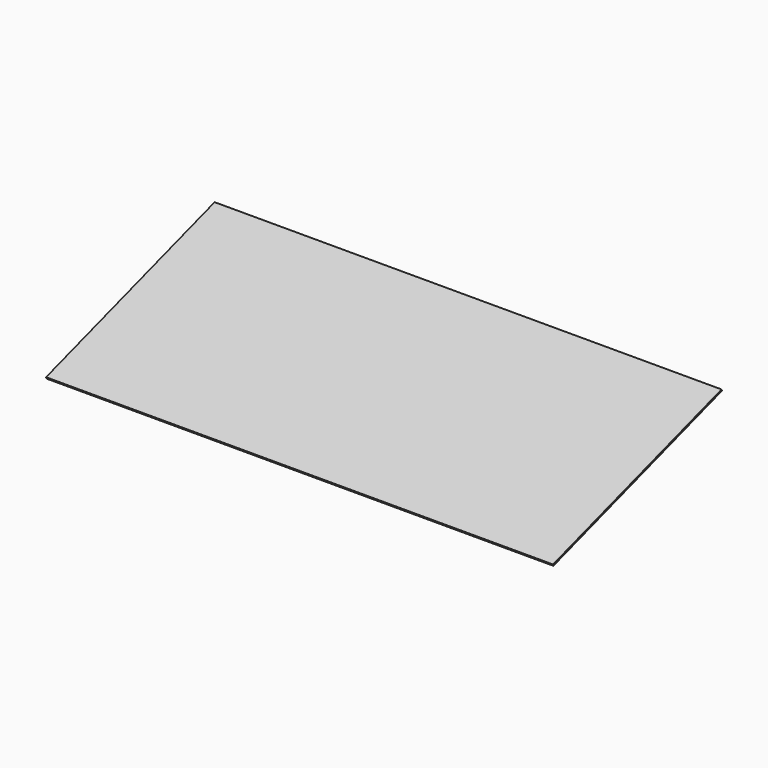
from build123d import *

# Parameters (mm, degrees)
F1_DEPTH = 550
F2_W     = 37.5
F2_H     = 447.9229075255
F3_DEPTH = 25


# Not quite as in the source:
# - a feature names something its author has since deleted; it is built from what else it names


with BuildPart() as f1:
    # F0 (on Right) → F1 (new body, symmetric)
    with BuildSketch(Plane.YZ):
        Polygon((1854.2745751406, 569.7310398559), (2042.2745751406, 630.8159427477), (2041.3475241575, 633.6691122966), (1853.3475241575, 572.5842094048), align=None)
        Polygon((2041.3475241575, 633.6691122966), (2042.2745751406, 630.8159427477), (2092.2745751406, 647.0619275593), (2091.3475241575, 649.9150971082), align=None)
        Polygon((2091.3475241575, 649.9150971082), (2092.2745751406, 647.0619275593), (2280.2745751406, 708.1468304511), (2279.3475241575, 711), align=None)
    extrude(amount=F1_DEPTH, both=True)

    # F2 (on face) → F3 (cut)
    with BuildSketch(Plane(origin=(0, 8.7006633238, -26.7778882743), x_dir=(1, 0, 0), z_dir=(0, -0.3090169944, 0.9510565163))):
        with Locations((-531.25, 2163.5379449891)):
            Rectangle(F2_W, F2_H)
        with Locations((531.25, 2163.5379449891)):
            Rectangle(F2_W, F2_H)
    extrude(amount=-F3_DEPTH, mode=Mode.SUBTRACT)


solid = f1.part
